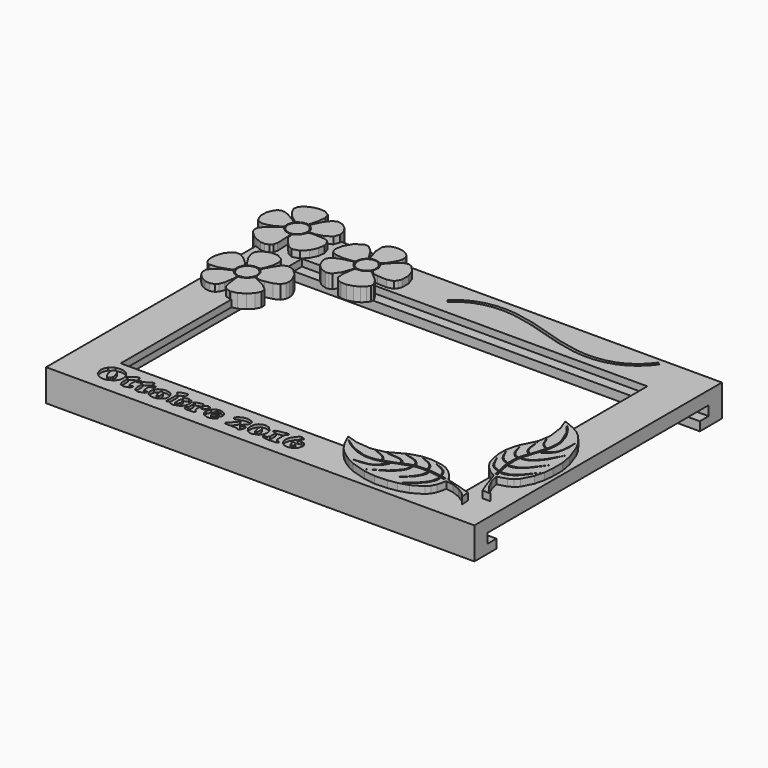
from build123d import *

# Parameters (mm, degrees)
F0_W      = 140.9999974
F0_H      = 92.0000192
F0_W_2    = 7
F1_DEPTH  = 2.5
F2_DEPTH  = 9
F3_DEPTH  = 2.3
F6_DEPTH  = 4
F5_W      = 4
F5_H      = 3.5
F7_DEPTH  = 4
F8_W      = 92.0000192
F8_H      = 3.5
F9_DEPTH  = 4
F11_DEPTH = 1
F12_DEPTH = 2.5
F13_DEPTH = 2.5
F14_DEPTH = 2


# Not quite as in the source:
# - ends of sketch curves that miss each other by under 0.0002 mm in the source are joined


with BuildPart() as f1:
    # F0 (on Top) → F1 (new body)
    with BuildSketch(Plane.XY):
        with Locations((19.9077800781, 3.6383251339)):
            Rectangle(F0_W, F0_H)
        Polygon((-42.5922186219, -37.3616844661), (-42.5922186219, 44.6383347339), (-42.3106248219, 44.6383347339), (82.4077787781, 44.6383347339), (82.4077787781, -37.3616844661), align=None, mode=Mode.SUBTRACT)
        Polygon((90.4077787781, -42.3616844661), (-50.5922186219, -42.3616844661), (-50.5922186219, 49.6383347339), (90.4077787781, 49.6383347339), (97.4077787781, 49.6383347339), (97.4077787781, 59.6383347339), (-57.5922186219, 59.6383347339), (-57.5922186219, -52.2210754661), (-57.5922186219, -52.3616844661), (-57.3105186219, -52.3616844661), (97.4077787781, -52.3616844661), (97.4077787781, -52.2210754661), (97.4077787781, -42.3616844661), align=None)
        with Locations((93.9077787781, 3.6383251339)):
            Rectangle(F0_W_2, F0_H)
    extrude(amount=F1_DEPTH)

    # F0 (on Top) → F2 (join)
    with BuildSketch(Plane.XY):
        Polygon((90.4077787781, -42.3616844661), (-50.5922186219, -42.3616844661), (-50.5922186219, 49.6383347339), (90.4077787781, 49.6383347339), (97.4077787781, 49.6383347339), (97.4077787781, 59.6383347339), (-57.5922186219, 59.6383347339), (-57.5922186219, -52.2210754661), (-57.5922186219, -52.3616844661), (-57.3105186219, -52.3616844661), (97.4077787781, -52.3616844661), (97.4077787781, -52.2210754661), (97.4077787781, -42.3616844661), align=None)
    extrude(amount=-F2_DEPTH)

    # F0 (on Top) → F3 (join)
    with BuildSketch(Plane.XY):
        with Locations((93.9077787781, 3.6383251339)):
            Rectangle(F0_W_2, F0_H)
    extrude(amount=-F3_DEPTH)

    # F4 (on face) → F6 (cut)
    with BuildSketch(Plane(origin=(0, -42.3616844661, 0), x_dir=(-1, 0, 0), z_dir=(0, 1, 0))):
        Polygon((54.5922186219, -2.3), (-97.4077787781, -2.3), (-97.4077787781, -5.8), (54.5728355646, -5.8), (54.5922186219, -5.8), align=None)
    extrude(amount=-F6_DEPTH, mode=Mode.SUBTRACT)

    # F5 (on face) → F7 (cut)
    with BuildSketch(Plane.XZ.offset(-49.6383347339)):
        with Locations((-52.5922186219, -4.05)):
            Rectangle(F5_W, F5_H)
        Polygon((97.4077787781, -5.8), (97.4077787781, -2.3), (90.4077787781, -2.3), (-50.5922186219, -2.3), (-50.5922186219, -5.8), align=None)
    extrude(amount=-F7_DEPTH, mode=Mode.SUBTRACT)

    # F8 (on face) → F9 (cut)
    with BuildSketch(Plane.YZ.offset(-50.5922186219)):
        with Locations((3.6383251339, -4.05)):
            Rectangle(F8_W, F8_H)
    extrude(amount=-F9_DEPTH, mode=Mode.SUBTRACT)

    # F10 (on face) → F11 (cut)
    with BuildSketch(Plane.XY.offset(2.5)):
        Polygon((-39.0562498219, -40.2667686661), (-40.3832982219, -40.0642036661), (-42.0479634219, -40.3508426661), (-43.8284018219, -41.6627272661), (-44.3864906219, -42.7431162661), (-44.5725202219, -43.9778356661), (-43.9937558219, -46.0448876661), (-42.3456260219, -47.4945926661), (-40.5210932219, -47.8914676661), (-39.0714136219, -47.6599466661), (-37.1697156219, -46.4086918661), (-36.5247842219, -45.3145360661), (-36.3098240219, -44.0825598661), (-36.7452816219, -42.3186822661), (-37.9083476219, -40.8744890661), align=None)
        Polygon((-41.6400648219, -42.0596022661), (-40.9069446219, -41.6461918661), (-40.3502274219, -41.8501538661), (-39.8651636219, -42.3793120661), (-39.3084210219, -43.6967084661), (-39.0934608219, -45.1353898661), (-39.3525154219, -45.9622106661), (-40.0250058219, -46.2764086661), (-40.5376286219, -46.1165410661), (-40.9565508219, -45.6865952661), (-41.5959704219, -44.2369156661), (-41.8495386219, -42.7927224661), align=None, mode=Mode.SUBTRACT)
        Polygon((-32.5560342219, -45.5598238661), (-32.5560342219, -43.6967084661), (-32.5009162219, -43.4872600661), (-32.2914678219, -43.4321420661), (-31.2937558219, -43.4321420661), (-31.0126286219, -43.3329042661), (-30.9354634219, -42.9635882661), (-30.9354634219, -42.6383920661), (-30.9960932219, -42.3241940661), (-31.2606850219, -42.2470288661), (-32.2804188219, -42.2470288661), (-32.5064280219, -42.1973972661), (-32.5560342219, -41.9824370661), (-32.5560342219, -41.2382932661), (-32.6056404219, -40.9902368661), (-32.7875552219, -40.9240952661), (-33.2340364219, -40.9240952661), (-33.4655320219, -40.9737014661), (-35.9901142219, -42.5612014661), (-36.1168856219, -42.8037460661), (-36.1168856219, -43.0462906661), (-36.0727912219, -43.2943216661), (-35.8688546219, -43.3439278661), (-35.3010884219, -43.3439278661), (-35.1467580219, -43.3769986661), (-35.1136872219, -43.5313544661), (-35.1136872219, -46.0779584661), (-34.5789918219, -47.3953802661), (-33.1623830219, -47.8914676661), (-31.2661968219, -47.2244890661), (-30.8913690219, -46.5685340661), (-31.0016050219, -46.2212906661), (-31.2441496219, -46.0614230661), (-31.4095036219, -46.1110292661), (-31.9772698219, -46.3094794661), (-32.3961920219, -46.1000056661), align=None)
        Polygon((-27.3305176219, -45.5598238661), (-27.3305176219, -43.6967084661), (-27.2753996219, -43.4872600661), (-27.0659258219, -43.4321420661), (-26.0682392219, -43.4321420661), (-25.7871120219, -43.3329042661), (-25.7099468219, -42.9635882661), (-25.7099468219, -42.6383920661), (-25.7705766219, -42.3241940661), (-26.0351684219, -42.2470288661), (-27.0549022219, -42.2470288661), (-27.2809114219, -42.1973972661), (-27.3305176219, -41.9824370661), (-27.3305176219, -41.2382932661), (-27.3801238219, -40.9902368661), (-27.5620386219, -40.9240952661), (-28.0085198219, -40.9240952661), (-28.2400154219, -40.9737014661), (-30.7645976219, -42.5612014661), (-30.8913690219, -42.8037460661), (-30.8913690219, -43.0462906661), (-30.8472746219, -43.2943216661), (-30.6433126219, -43.3439278661), (-30.0755718219, -43.3439278661), (-29.9212414219, -43.3769986661), (-29.8881452219, -43.5313544661), (-29.8881452219, -46.0779584661), (-29.3534752219, -47.3953802661), (-27.9368664219, -47.8914676661), (-26.0406802219, -47.2244890661), (-25.6658524219, -46.5685340661), (-25.7760884219, -46.2212906661), (-26.0186330219, -46.0614230661), (-26.1839870219, -46.1110292661), (-26.7517532219, -46.3094794661), (-27.1706754219, -46.1000056661), align=None)
        Polygon((-20.2529092219, -42.7706752661), (-22.0223240219, -42.2470288661), (-23.3631392219, -42.4647576661), (-24.4862510219, -43.1179440661), (-25.2138594219, -44.0632812661), (-25.4563786219, -45.2456258661), (-25.2579538219, -46.3039676661), (-24.6626286219, -47.1418120661), (-23.7214316219, -47.7040410661), (-22.5294350219, -47.8914676661), (-21.2547360219, -47.6916458661), (-20.1316496219, -47.0922058661), (-19.3089690219, -46.1647756661), (-19.0347252219, -45.0582246661), (-19.3764822219, -43.7463146661), align=None)
        Polygon((-22.8546566219, -43.7022202661), (-22.4632934219, -43.5203308661), (-21.9561570219, -43.9061822661), (-21.6585198219, -44.8652862661), (-21.5317230219, -45.9181162661), (-21.6543796219, -46.3852730661), (-22.0223240219, -46.5409750661), (-22.5790412219, -46.0889820661), (-22.8767038219, -45.0802718661), (-22.9979634219, -44.1762604661), align=None, mode=Mode.SUBTRACT)
        Polygon((-15.7053948219, -42.6990218661), (-15.6337414219, -40.5492674661), (-15.9203550219, -40.2185340661), (-17.0227912219, -40.3618662661), (-18.0921566219, -40.6870878661), (-18.8803948219, -41.4091590661), (-18.7701334219, -41.7123334661), (-18.3732584219, -41.9493662661), (-18.1252274219, -42.1753500661), (-18.0811330219, -42.8864230661), (-18.0811330219, -44.4077814661), (-18.1197156219, -46.0834702661), (-18.2685342219, -46.9709208661), (-18.2960932219, -47.1363002661), (-17.9543362219, -47.3567722661), (-17.6181164219, -47.3016542661), (-17.2763594219, -47.1969300661), (-17.1440508219, -47.2465362661), (-16.1408524219, -47.7426236661), (-15.1045578219, -47.8914676661), (-13.0871120219, -47.1969300661), (-12.1900094219, -46.0765868661), (-11.8909752219, -44.6337906661), (-12.0756332219, -43.6154030661), (-12.6296072219, -42.8092578661), (-13.9910980219, -42.2525406661), (-15.4132440219, -42.7816988661), (-15.6337414219, -42.9305174661), (-15.7053948219, -42.8202814661), align=None)
        Polygon((-15.5896216219, -44.1156306661), (-15.1596758219, -43.9116940661), (-14.6691002219, -44.1762604661), (-14.3163196219, -45.5763592661), (-14.5257934219, -46.5685340661), (-15.1376286219, -46.9102910661), (-15.6061570219, -46.4913688661), (-15.6943712219, -44.7440266661), align=None, mode=Mode.SUBTRACT)
        Polygon((-8.5616448219, -42.3682884661), (-8.9144254219, -42.2856114661), (-10.3585932219, -42.5446660661), (-11.2626046219, -42.9250056661), (-11.5326828219, -43.3769986661), (-11.1413196219, -43.8235052661), (-10.9208476219, -43.9998828661), (-10.8657296219, -44.3526634661), (-10.9539184219, -46.2102670661), (-11.0365954219, -46.4472744661), (-11.2570928219, -46.6347010661), (-11.5878008219, -47.1473238661), (-11.1358078219, -47.6819938661), (-9.6530320219, -47.8528850661), (-8.0986282219, -47.7426236661), (-7.6741688219, -47.5221516661), (-7.5143266219, -47.1252766661), (-8.0104140219, -46.6071420661), (-8.3080766219, -46.4803452661), (-8.4128008219, -46.2488496661), (-8.4734560219, -45.1133426661), (-8.4293362219, -44.3857342661), (-8.2253996219, -44.2093566661), (-8.0104140219, -44.3251044661), (-7.5143266219, -44.7274912661), (-7.0402864219, -44.8267036661), (-6.1748830219, -44.4904584661), (-5.8606850219, -44.0439772661), (-5.7394254219, -43.5093072661), (-5.8386378219, -43.0297552661), (-6.0922060219, -42.6163194661), (-6.9135150219, -42.2911232661), (-8.0655320219, -42.9801236661), (-8.2750058219, -43.1399912661), (-8.4458716219, -42.8974466661), align=None)
        Polygon((-3.0439774219, -45.2731848661), (-0.4532536219, -45.2731848661), (-0.0674022219, -45.0472010661), (0.0814163781, -44.4573876661), (-0.1776636219, -43.5534016661), (-0.7729634219, -42.8478404661), (-2.5534018219, -42.2525406661), (-3.7715858219, -42.4895480661), (-5.0063052219, -43.4431656661), (-5.5685342219, -45.1078308661), (-5.2433126219, -46.4197154661), (-4.6149420219, -47.2189772661), (-2.6746614219, -47.8914676661), (-0.6517038219, -47.2355126661), (-0.1556164219, -46.4693216661), (-0.2934114219, -46.1055174661), (-0.5745386219, -45.9291398661), (-0.8721758219, -46.0614230661), (-1.4068712219, -46.3149912661), (-1.9911474219, -46.4142036661), (-2.8289918219, -46.1000056661), (-3.2148432219, -45.4220288661), align=None)
        Polygon((-2.3439280219, -44.2424274661), (-2.9006452219, -44.2424274661), (-3.1817724219, -44.1762604661), (-3.2589376219, -43.9447648661), (-3.0935836219, -43.4872600661), (-2.6085198219, -43.2447154661), (-2.1620386219, -43.4321420661), (-1.9911474219, -43.9172058661), align=None, mode=Mode.SUBTRACT)
        Polygon((3.6698267781, -47.7426236661), (7.4236165781, -47.7426236661), (7.7763717781, -47.7867434661), (7.9748219781, -47.9851682661), (8.1622231781, -48.2001538661), (8.3827205781, -48.2607836661), (9.0111165781, -47.9300502661), (9.4355505781, -47.1969300661), (9.5953927781, -46.3590856661), (9.4741331781, -45.7389700661), (9.1103289781, -45.5322648661), (8.9339259781, -45.5708474661), (8.6803831781, -45.7968566661), (7.8149797781, -46.1716590661), (7.4677109781, -46.0669348661), (7.3243787781, -45.8023684661), (7.7984189781, -45.2070432661), (8.7988995781, -44.1183992661), (9.1323761781, -43.1124322661), (8.9339259781, -42.3848238661), (8.4102795781, -41.8446420661), (6.5857467781, -41.4201826661), (5.2008371781, -41.6337966661), (3.9454421781, -42.2745878661), (3.4217703781, -42.7927224661), (3.2233455781, -43.2777862661), (3.4383311781, -43.7187556661), (3.9178831781, -43.9172058661), (4.2375929781, -43.8179934661), (4.8218691781, -43.3714868661), (5.2077205781, -43.2998334661), (5.6376663781, -43.4652128661), (5.7975085781, -43.9006704661), (5.5329421781, -44.6613496661), (3.9564657781, -46.5299514661), (3.2784635781, -47.1969300661), (3.1737393781, -47.4615218661), align=None)
        Polygon((14.5673665781, -41.7509160661), (13.1121497781, -41.3816000661), (11.9807829781, -41.5759100661), (11.0561213781, -42.1588146661), (10.3574435781, -43.2006210661), (10.1245509781, -44.5731354661), (10.3794907781, -45.9911412661), (11.1443101781, -47.0922058661), (12.0951591781, -47.6916458661), (13.2278975781, -47.8914676661), (15.2012489781, -47.1748828661), (16.0487453781, -46.0986340661), (16.3312441781, -44.7550502661), (15.9839753781, -43.2281800661), align=None)
        Polygon((12.6008985781, -43.2419722661), (12.9853783781, -43.0242434661), (13.4869775781, -43.4321420661), (13.7570811781, -44.3526634661), (13.8673171781, -45.4110052661), (13.7419173781, -46.0765868661), (13.3657179781, -46.2984558661), (12.9081877781, -45.9456752661), (12.4727301781, -43.8951586661), align=None, mode=Mode.SUBTRACT)
        Polygon((17.5439163781, -46.7063544661), (17.1801121781, -46.6677718661), (16.8383551781, -46.7945432661), (16.7005601781, -47.0811822661), (17.1249941781, -47.5441988661), (18.3486899781, -47.8143024661), (19.6826217781, -47.8969794661), (21.7772581781, -47.7150646661), (22.5103783781, -47.1638592661), (21.9922183781, -46.7394252661), (21.3528241781, -46.6071420661), (21.1047677781, -46.2047552661), (21.0606733781, -45.9126044661), (21.0110671781, -44.3306162661), (21.0882323781, -42.6549274661), (21.4795955781, -42.2911232661), (21.7662345781, -42.1202320661), (21.8378879781, -41.8942482661), (21.6173905781, -41.5359558661), (20.9228783781, -41.4202080661), (17.6045461781, -42.0816494661), (17.1139705781, -42.3903356661), (16.9375929781, -42.7376044661), (17.0533407781, -43.0077080661), (17.3565151781, -43.1069204661), (17.5494281781, -43.0958714661), (17.7699255781, -43.0793360661), (18.2108949781, -43.1951092661), (18.3321545781, -43.6085196661), (18.2935719781, -45.9897696661), (17.7533901781, -46.7284016661), align=None)
        Polygon((26.1924893781, -40.7422058661), (25.4152747781, -40.5713146661), (24.8364849781, -40.8579536661), (23.9876169781, -41.8336184661), (23.1484009781, -43.2777862661), (22.8686453781, -44.6889086661), (23.0946545781, -45.8740218661), (23.8608455781, -47.0536232661), (24.8943715781, -47.6819938661), (26.2090247781, -47.8914676661), (27.7455469781, -47.5455704661), (28.8493547781, -46.5079042661), (29.3344185781, -44.9314278661), (29.1345967781, -43.9998828661), (28.5351567781, -43.2777862661), (27.2728783781, -42.8368168661), (26.4129613781, -43.0021708661), (26.0160863781, -43.1234558661), (25.8948267781, -43.0683378661), (25.8452205781, -42.9250056661), (26.0160863781, -42.4178946661), (26.4129613781, -41.8446420661), (26.8153481781, -41.3760882661), (26.8815151781, -41.2052224661), (26.6830649781, -40.9681896661), align=None)
        Polygon((25.6302349781, -44.5731354661), (26.0160863781, -44.3967578661), (26.4129613781, -44.5455764661), (26.8153481781, -45.1409016661), (26.9807275781, -45.9070926661), (26.8429071781, -46.2653850661), (26.4791283781, -46.3976682661), (25.8176615781, -45.9511870661), (25.4924399781, -45.0416892661), align=None, mode=Mode.SUBTRACT)
        Polygon((76.7236557781, 57.2223175339), (75.7524359781, 57.8975511339), (73.8715151781, 55.5857955339), (71.6687509781, 53.5751315339), (69.1965689781, 51.9068087339), (66.5074455781, 50.6220513339), (63.2374749781, 49.6519237339), (59.8428157781, 49.1732353339), (56.3862313781, 49.1225369339), (52.9304597781, 49.4364047339), (46.1256219781, 50.8679233339), (39.3970095781, 52.8715769339), (32.6121615781, 54.8672803339), (25.6447383781, 56.2565841339), (22.0671229781, 56.5266877339), (18.4725403781, 56.4069013339), (14.9295197781, 55.8262319339), (11.5066411781, 54.7137373339), (8.1951923781, 52.9586227339), (5.2492241781, 50.6419141339), (6.0611859781, 49.7814637339), (8.8406317781, 51.9669305339), (11.9646793781, 53.6228835339), (15.2065575781, 54.6750785339), (18.5874753781, 55.2281127339), (22.0405037781, 55.3435811339), (25.4986883781, 55.0830533339), (32.3128987781, 53.7218419339), (39.0447877781, 51.7421405339), (45.8184851781, 49.7243137339), (52.7684077781, 48.2645249339), (56.3391651781, 47.9396843339), (59.9332397781, 47.9921353339), (63.4865981781, 48.4944203339), (66.9351815781, 49.5190817339), (69.7845027781, 50.8796073339), (72.4008297781, 52.6446279339), (74.7314575781, 54.7726907339), align=None)
    extrude(amount=-F11_DEPTH, mode=Mode.SUBTRACT)

    # F10 (on face) → F12 (join)
    with BuildSketch(Plane.XY.offset(2.5)):
        Polygon((82.4077787781, -24.8222918728), (82.4077787781, -26.6389711426), (83.5959051781, -27.6658794661), (85.6334931781, -28.8352954661), (87.3536573781, -34.0525824661), (88.8356203781, -37.9930876661), (91.8024165781, -38.0176748661), (90.1737685781, -36.8249162661), (88.5281025781, -34.5089188661), (87.2255143781, -31.6619344661), (86.6260997781, -28.8761386661), (89.8929969781, -27.9246038661), (91.4917237781, -26.9786316661), (92.7525035781, -25.7694392661), (94.7395455781, -21.8603792661), (95.6326857781, -18.3121008661), (95.9526241781, -15.0635424661), (95.9534877781, -10.5948696661), (95.1512541781, -6.4291426661), (93.2918471781, -1.1702758661), (92.0235743781, 1.1986551339), (90.3933007781, 3.4321279339), (88.7402433781, 5.2896553339), (87.1759843781, 6.5801277339), (84.6684455781, 8.0475619339), (82.4077787781, 8.9595404574), (82.4077787781, 8.3104146703), (84.4963351781, 6.1215307339), (86.1499005781, 3.5666209339), (87.1506859781, 1.4285505339), (87.9832979781, -1.5905950661), (88.0010525781, -4.5525652661), (87.3128395781, -8.3344220661), (86.2622701781, -10.8951738661), (84.7916355781, -15.7043590661), (84.5624513781, -18.1463658661), (84.8761921781, -22.3070382661), (86.0933347781, -27.5964866661), (85.3364147781, -27.6957498661), (84.2792921781, -22.8573800661), (83.9435803781, -20.3930720661), (83.9373319781, -17.8612254661), (84.0348171781, -16.1369210661), (84.5069523781, -14.1969706661), (85.9491643781, -10.3173746661), (86.93214141, -6.8113595297), (85.8107597781, -6.3159856661), (84.8599869781, -5.5106532661), (84.1876743781, -4.4411100661), (83.0931883781, -1.6576510661), (83.9026609781, -3.1752502661), (84.6109907781, -4.7800984661), (85.5973489781, -5.8532992661), (86.9969143781, -6.4533996661), (86.9495239967, -6.7493605105), (87.3466469781, -5.3329294661), (87.5562223781, -2.9158908661), (87.3419733781, -0.6577292661), (85.3261531781, 4.3245061339), (82.4077787781, 8.2377713206), (82.4077787781, 4.2659286823), (82.9804377781, 0.0068363339), (82.4077787781, -3.6377173348), (82.4077787781, -14.9819990927), (83.7716985781, -15.8728372661), (83.7145485781, -16.3442358661), (82.4425927781, -15.4811438661), (82.4077787781, -15.4407730706), (82.4077787781, -19.7287612836), (83.6703271781, -20.2725490661), (83.7088589781, -20.6955098661), (82.4077787781, -20.1635944295), (82.4077787781, -24.4548522413), (82.5383761781, -24.5969498661), (84.3776155781, -25.3688558661), (84.3728403781, -25.8263860661), (82.7927063781, -25.1483330661), align=None)
        Polygon((86.3122065781, -26.4910024661), (86.2192425781, -26.0206706661), (88.9610709781, -25.3765266661), (90.9982779781, -23.9398772661), (95.1068295781, -18.9487010661), (91.8285785781, -23.5265430661), (90.3175833781, -25.0708122661), (88.4368403781, -26.0726136661), (87.3511427781, -26.4410660661), align=None, mode=Mode.SUBTRACT)
        Polygon((85.2411647781, -21.7964474661), (85.2425871781, -21.4030268661), (87.9522083781, -20.6377502661), (90.2719395781, -18.7704438661), (94.6556239781, -13.1043134661), (91.1733093781, -18.1236074661), (89.5136225781, -20.0028264661), (87.4600833781, -21.3564686661), (86.3037991781, -21.7672628661), (85.1797729781, -21.8577630661), align=None, mode=Mode.SUBTRACT)
        Polygon((83.7255721781, -10.8170434661), (84.9285669781, -11.8759440661), (84.7747699781, -12.2748256661), (83.7241497781, -11.3737098661), (83.0639783781, -10.0839232661), (82.8124421781, -8.6356406661), (82.4822675781, -5.1122034661), (82.8942555781, -7.2103958661), (83.0841713781, -9.2173514661), align=None, mode=Mode.SUBTRACT)
        Polygon((85.2076367781, -16.1215032661), (85.3454317781, -15.6061880661), (86.4809387781, -15.4454822661), (87.7624449781, -14.9350184661), (89.7831419781, -13.1407624661), (91.1158291781, -11.3798566661), (94.1942329781, -5.9575154661), (91.7894117781, -10.8244348661), (91.2931211781, -11.7546590661), (89.7832181781, -13.7347922661), (88.2971657781, -15.1115484661), (86.8241181781, -15.7740058661), align=None, mode=Mode.SUBTRACT)
        Polygon((87.3097915781, -9.6943888661), (87.4949067781, -9.0630210661), (89.7755473781, -7.2778328661), (90.5238821781, -6.1284828661), (91.0172771781, -4.6301876661), (91.3649269781, 0.9116097339), (91.4948225781, -2.3485564661), (91.1874317781, -4.9346574661), (90.6404935781, -6.5659216661), (89.2364831781, -8.4606346661), align=None, mode=Mode.SUBTRACT)
        Polygon((39.842011439, -37.3616844661), (39.2524704085, -37.3616844661), (40.3360729781, -39.7125152661), (41.9232681781, -42.1460130661), (43.2880101781, -43.6459084661), (45.2234393781, -45.2070432661), (47.5332645781, -46.7271824661), (49.9608695781, -47.8791994661), (55.3036579781, -49.4816346661), (59.5033447781, -50.0810746661), (63.9667597781, -49.8637014661), (67.1959887781, -49.3867402661), (70.6968453781, -48.3227342661), (74.5050165781, -46.1486212661), (75.6517249781, -44.8307422661), (76.5191095781, -43.1880480661), (77.3112593781, -39.8788852661), (80.1228107781, -40.3426130661), (83.0295867781, -41.5057298661), (85.4225969781, -43.0372736661), (86.6928509781, -44.6062062661), (86.5245251781, -41.6441090661), (82.5168623781, -40.3547796661), (77.2223339781, -38.8894282661), (76.2442013792, -37.3616844661), (73.9537955395, -37.3616844661), (74.1559189781, -37.7760446661), (73.6991253781, -37.8029940661), (73.4882151037, -37.3616844661), (64.4903989403, -37.3616844661), (64.6529915781, -37.5779500661), (64.1849203781, -37.6578838661), (63.9702919636, -37.3616844661), (58.6565628279, -37.3616844661), (59.6887647781, -37.8283686661), (60.6397153781, -38.8340816661), (60.2487839781, -39.0070302661), (59.1328095781, -37.8567658661), (57.7008650039, -37.3616844661), (49.6138425534, -37.3616844661), (48.2855363781, -37.6369288661), (45.0622309962, -37.3616844661), (39.8848763277, -37.3616844661), (44.0866115781, -40.1890954661), (49.1606679781, -41.9611518661), (51.4265511781, -42.0657236661), (53.8305849781, -41.7392828661), (55.2260700221, -41.2740153251), (54.9327925781, -41.3356768661), (54.2655853781, -39.9668454661), (53.1458517781, -39.0336494661), (51.5085931781, -38.4038818661), (49.9535289781, -37.6689074661), (52.7867465781, -38.6272494661), (53.8876333781, -39.2469586661), (54.7380761781, -40.1575740661), (55.2872144471, -41.2536292118), (58.7414717781, -40.1019480661), (62.5466457781, -38.4734270661), (64.4614501781, -37.9078960661), (66.1789981781, -37.7269718661), (68.7081523781, -37.6105382661), (71.1858461781, -37.8264382661), (76.0697581781, -38.6478996661), (76.0072741781, -39.4087312661), (70.6650699781, -38.4493224661), (66.4940851781, -38.3375370661), (64.0660483781, -38.6847550661), (59.3337743781, -40.3867074661), (56.8269213781, -41.5601112661), (53.0828597781, -42.4307470661), (50.1235057781, -42.5565024661), (47.0675555781, -41.8711596661), (44.8835365781, -40.9751492661), (42.2514869781, -39.4473138661), align=None)
        Polygon((55.8909059781, -44.0711044661), (57.5634959781, -41.7066438661), (58.1851609781, -41.4911502661), (57.0461741781, -43.4753728661), (55.2217175781, -44.9695278661), (53.6188759781, -45.5948504661), (51.0507073781, -46.0271838661), (47.7880773781, -46.0554032661), (53.3065321781, -45.4396564661), (54.7791733781, -44.8742524661), align=None, mode=Mode.SUBTRACT)
        Polygon((63.8893151781, -40.3846246661), (63.9948267781, -39.2426914661), (64.5028775781, -39.0800806661), (64.2340947781, -40.7114972661), (63.6437987781, -42.2148978661), (62.3406517781, -43.7659234661), (60.4359819781, -45.3699842661), (59.5309037781, -45.9107756661), (54.7862345781, -48.5485656661), (60.0530515781, -45.2110564661), (61.7473077781, -43.7946254661), (63.4415385781, -41.6893464661), align=None, mode=Mode.SUBTRACT)
        Polygon((69.1467595781, -41.6026054661), (69.7798799781, -38.8590752661), (70.1727417781, -38.8386028661), (70.2310347781, -38.7743154661), (70.1950937781, -39.9013896661), (69.8408145781, -41.0762412661), (68.5882389781, -43.1929502661), (66.7916461781, -44.9417148661), (61.9469771781, -48.6631450661), (67.3940579781, -44.0100682661), align=None, mode=Mode.SUBTRACT)
        Polygon((73.9288683781, -42.3806836661), (74.4394337781, -39.6108644661), (74.9137025781, -39.6809176661), (74.9141597781, -40.7210730661), (74.5987425781, -41.8233568661), (73.6892447781, -43.7504040661), (72.2199817781, -45.3344496661), (67.8063761781, -48.8306580661), (72.5925997781, -44.4850990661), align=None, mode=Mode.SUBTRACT)
        Polygon((-12.9422558219, 45.8867801339), (-10.8253944219, 46.4736725339), (-10.0408900219, 47.3849991339), (-9.5741142219, 48.5860889339), (-9.5298166219, 51.4818413339), (-10.5647396219, 54.4096993339), (-12.5510958219, 56.6184071339), (-13.9618880219, 57.1482765339), (-15.4609452219, 56.8088309339), (-17.2068650219, 55.5205175339), (-19.3582704219, 53.2037581339), (-20.0420892219, 52.2600211339), (-19.7511322219, 51.6057171339), (-19.0960408219, 49.9026471339), (-19.2493298219, 48.0996789339), (-19.3409222219, 47.4934571339), (-18.6529124219, 46.8839333339), (-17.7361756219, 46.3085979339), (-16.4363814219, 46.0565791339), align=None)
        Polygon((-45.6112278219, 43.7100763339), (-43.0470470219, 44.4288455339), (-41.2036420219, 46.3593725339), (-40.0380614219, 48.8445593339), (-39.7090298219, 51.3540539339), (-40.3751702219, 53.3576313339), (-41.2208124219, 54.0539469339), (-42.5364562219, 54.4803113339), (-47.0275572219, 54.6075399339), (-48.2771610219, 54.3081247339), (-48.4021544219, 53.6125965339), (-49.2000192219, 52.0704355339), (-50.5825158219, 51.0020607339), (-51.0287430219, 50.6574589339), (-50.9266350219, 49.5753173339), (-50.6253910219, 48.5030055339), (-49.5220658219, 46.9481445339), (-47.4045694219, 44.6375319339), align=None)
        Polygon((-42.5922186219, 32.3775420091), (-42.5922186219, 23.9327596608), (-41.9784944219, 23.6751151339), (-40.8202798219, 23.3489537339), (-39.2281570219, 23.4811861339), (-36.5299150219, 24.0420943339), (-34.6559792219, 24.9394509339), (-33.7853942219, 26.3138957339), (-33.5992884219, 27.7198111339), (-33.8199382219, 29.2090893339), (-35.2165572219, 32.0742855339), (-37.4454072219, 34.1825871339), (-38.7063648219, 34.7257661339), (-39.9766696219, 34.8071731339), (-40.9658472219, 34.3986903339), (-41.9755226219, 33.4303661339), align=None)
        Polygon((-26.7615830219, 49.0437969339), (-26.7513214219, 49.4374715339), (-26.3703722219, 51.0412783339), (-25.4230792219, 52.3593097339), (-25.0174920219, 52.7854455339), (-27.5075302219, 56.7626029339), (-29.5965532219, 58.5955685339), (-30.6243134219, 58.7672725339), (-31.7499398219, 58.4868057339), (-33.9363210219, 56.7792145339), (-35.4245832219, 54.1863063339), (-35.9222200219, 51.4875055339), (-35.7081488219, 50.3419909339), (-35.1366996219, 49.4622873339), (-33.6582926219, 48.8117933339), (-31.0597710219, 48.5155531339), (-28.0792334219, 48.7788749339), align=None)
        Polygon((-16.5280514482, 44.6383347339), (-24.1622243817, 44.6383347339), (-24.2788600219, 44.1817035339), (-24.7316658219, 40.5974079339), (-24.4898578219, 38.2244383339), (-23.5451810219, 37.0614993339), (-21.9679426219, 36.4446857339), (-19.9640350219, 36.4113609339), (-17.7393252219, 36.9989137339), (-16.0075532219, 37.9037125339), (-14.7289680219, 39.0003321339), (-13.9946286219, 40.1855215339), (-13.8956702219, 41.3559789339), (-15.2740774219, 43.5413949339), align=None)
        Polygon((-45.0493544219, 28.8051785339), (-44.3935518219, 29.9630629339), (-43.5239828219, 32.4943761339), (-43.2844100219, 35.0165199339), (-43.5431344219, 36.1768173339), (-44.1697016219, 37.1228911339), (-46.2241806219, 38.2921801339), (-48.8436064219, 38.3639351339), (-51.4237130219, 37.1777551339), (-52.4950088219, 35.8463633339), (-52.6268348219, 34.1469509339), (-51.7846978219, 31.8870367339), (-49.9340284219, 28.8741141339), (-49.3335724219, 28.1330183339), (-48.7411174219, 28.3608817339), (-47.2852148219, 28.9154399339), (-45.7747530219, 28.8153639339), align=None)
        Polygon((-57.5922186219, 59.6383347339), (-50.9054715871, 59.6383347339), (-50.4340782219, 61.3726013339), (-50.0464742219, 64.5712487339), (-50.7474126219, 66.5318239339), (-52.6481708219, 67.6120859339), (-54.3338672219, 67.7605743339), (-56.1619306219, 67.5033231339), (-57.9087648219, 66.8944851339), (-59.3508498219, 65.9881877339), (-60.4002000219, 64.6763285339), (-60.5203166219, 63.2179875339), (-59.6810244219, 61.4789257339), (-57.8520974219, 59.3249041339), (-57.5922186219, 59.1312214795), align=None)
        Polygon((-50.6763180219, 12.9225839339), (-49.1059376219, 13.4136929339), (-48.2846032219, 14.3361701339), (-47.6314676219, 15.8664439339), (-47.0996170219, 19.8809901339), (-47.1866120219, 20.9995299339), (-47.6864586219, 21.2600323339), (-49.1985460219, 22.1203811339), (-50.1070278219, 23.2538053339), (-53.1745350219, 21.8660763339), (-55.4472508219, 20.2756299339), (-56.5987090219, 18.7598341339), (-56.6763060219, 17.2002487339), (-55.7273366219, 15.4783827339), (-54.1916018219, 14.0187209339), (-52.4397384219, 13.1455197339), align=None)
        Polygon((-57.5922186219, 31.4267985945), (-57.5922186219, 21.8893522871), (-55.1119454219, 21.9585069339), (-51.5761892219, 23.1175089339), (-50.3858690219, 23.7181935339), (-50.4540934219, 24.0407481339), (-50.4940222219, 25.6275623339), (-49.9720522219, 27.0809503339), (-49.6713416219, 27.8114035339), (-50.3536872219, 28.6524737339), (-52.9271390219, 30.9995607339), (-54.9885014219, 32.2009807339), (-56.5233726219, 32.1426369339), align=None)
        Polygon((-57.5922186219, 51.3998818667), (-57.5922186219, 42.5509348584), (-55.0931748219, 41.5467583339), (-53.5318876219, 41.4714981339), (-52.1617862219, 41.8799809339), (-51.4085238219, 42.7045157339), (-51.0063148219, 44.1962323339), (-51.2237642219, 49.4341441339), (-51.4301646219, 50.5517187339), (-52.0319668219, 50.6692191339), (-53.7630276219, 51.0756445339), (-55.1487500219, 52.1977403339), (-55.6524320219, 52.6539243339), (-56.5192324219, 52.2027441339), align=None)
        Polygon((-58.3444510219, 51.6291867339), (-57.5922186219, 52.0513407308), (-57.5922186219, 58.3858754724), (-59.6399272219, 59.6188583339), (-61.3068784219, 60.2213971339), (-62.5030406219, 60.3216509339), (-63.4289214219, 59.9007475339), (-64.1911754219, 59.1213993339), (-65.1491618219, 56.8456863339), (-65.2259460219, 54.2112745339), (-64.2704996219, 51.9348757339), (-63.2895262219, 51.1112553339), (-62.0419798219, 50.7892341339), (-60.4271748219, 50.9636051339), align=None)
        Polygon((57.8984965781, -33.8612188661), (57.4105130467, -34.1479347624), (61.1516269781, -34.9136424661), (62.5609713781, -35.4366538661), (63.7292697781, -36.3493012661), (64.4903989403, -37.3616844661), (73.4882151037, -37.3616844661), (72.8390305781, -36.0033278661), (71.5046669781, -34.8912396661), (67.4043703781, -33.0260922661), (71.0767277781, -34.4069632661), (72.3886123781, -35.1454428661), (73.4020723781, -36.2306324661), (73.9537955395, -37.3616844661), (76.2442013792, -37.3616844661), (75.9555851781, -36.9108952661), (74.0932571781, -34.9562128661), (71.9553645781, -33.5183442661), (70.1352259781, -32.8479112661), (65.8778303781, -32.2251540661), (62.6639429781, -32.3724740661), (59.5175941781, -33.2198434661), align=None)
        Polygon((68.9988807781, -37.3614404661), (68.5745483781, -37.3434318661), (67.6951749781, -35.5467882661), (66.3608367781, -34.4347000661), (62.2605147781, -32.5695526661), (65.9328975781, -33.9503982661), (67.2447821781, -34.6889032661), (68.2582421781, -35.7740674661), align=None, mode=Mode.SUBTRACT)
        Polygon((-17.1355418219, 59.4965065339), (-17.1987458467, 59.6383347339), (-26.3000436102, 59.6383347339), (-26.1513480219, 57.3544737339), (-24.7713152219, 53.1033773339), (-23.8809182219, 53.1392675339), (-22.4583404219, 53.2709157339), (-20.6316232219, 52.5433835339), (-19.4514884219, 53.5864091339), (-17.5761048219, 56.7306497339), (-17.1438222219, 58.2442103339), align=None)
        Polygon((-42.5922186219, 23.5646985702), (-42.5922186219, 12.7591575143), (-40.7447402219, 13.1467897339), (-38.4791618219, 14.4738635339), (-36.7853374219, 16.2073373339), (-35.8998934219, 18.0218371339), (-36.0594054219, 19.5918873339), (-38.4518822219, 21.6099427339), align=None)
        Polygon((-24.5177990244, 44.6383347339), (-34.3742825943, 44.6383347339), (-34.3564116219, 43.6538407339), (-33.2915166219, 41.1643359339), (-31.3772456219, 39.3722643339), (-29.1648548219, 38.6178589339), (-28.1191368219, 38.7360959339), (-27.2056766219, 39.2413019339), (-25.6360582219, 41.5119603339), (-24.5358572219, 44.5489875339), align=None)
        Polygon((81.5532879781, -25.9004270661), (82.4077787781, -26.6389711426), (82.4077787781, -24.8222918728), (81.6596885781, -24.1886448661), (80.8585217781, -22.9140728661), (79.3013493781, -19.3129116661), (81.3629657781, -23.3180344661), (82.4077787781, -24.4548522413), (82.4077787781, -20.1635944295), (82.0874753781, -20.0326460661), (80.9544575781, -19.0729578661), (80.1532653781, -17.7983858661), (78.5960929781, -14.1972500661), (80.6577347781, -18.2023728661), (81.8331451781, -19.4812628661), (82.4077787781, -19.7287612836), (82.4077787781, -15.4407730706), (81.4744209781, -14.3584384661), (80.8837185781, -12.9760942661), (79.9376672282, -9.2764421595), (79.6749325781, -9.7777516661), (79.1127543781, -11.4260084661), (78.4188263781, -14.6097460661), (78.4273861781, -17.8269862661), (79.2557055781, -22.0492282661), (80.0135145781, -23.8347212661), align=None)
        Polygon((-22.4276318219, 45.8098181339), (-20.7618744219, 46.5203831339), (-19.8811294219, 47.4809603339), (-19.4427762219, 48.5872065339), (-19.7178074219, 50.8501179339), (-21.2359146219, 52.5361445339), (-22.3514572219, 52.9212593339), (-23.6461206219, 52.8722627339), (-24.9566844219, 52.3235211339), (-25.8678840219, 51.3851943339), (-26.3249570219, 50.1445059339), (-26.2731410219, 48.6887049339), (-25.4701200219, 47.0068439339), (-24.0926780219, 46.0095891339), align=None)
        Polygon((-51.9848244219, 50.9922817339), (-50.8660306219, 51.2243869339), (-49.2983172219, 52.4671581339), (-48.6363932219, 54.2201645339), (-48.9241498219, 56.0613343339), (-50.2055798219, 57.5686211339), (-51.9661808219, 58.1680357339), (-53.6733148219, 57.8231037339), (-55.0039446219, 56.6909241339), (-55.6350838219, 54.9285705339), (-55.4441520219, 53.4076185339), (-54.6840570219, 52.1496327339), (-53.4869296219, 51.2970309339), align=None)
        Polygon((-47.0697720219, 21.4676773339), (-45.1469158219, 21.8082405339), (-43.6980490219, 23.1316059339), (-43.1749614219, 24.9004365339), (-43.5899974219, 26.7058177339), (-44.9555268219, 28.1389365339), (-46.5835144219, 28.6109447339), (-48.1943316219, 28.2676383339), (-49.4921954219, 27.2476251339), (-50.1812720219, 25.6895383339), (-49.9471094219, 23.6860117339), (-48.7898854219, 22.1861671339), align=None)
        Polygon((-40.3657468219, 59.0512953339), (-40.466210318, 59.6383347339), (-50.2205466938, 59.6383347339), (-50.8535592219, 58.3767983339), (-50.2247060219, 57.9356003339), (-49.0452062219, 56.8979849339), (-48.4493730219, 55.5447237339), (-48.1579080219, 54.9530307339), (-47.0107170219, 54.9382987339), (-45.8888498219, 54.9711663339), (-43.2962464219, 55.7267147339), (-41.1317346219, 57.0936665339), align=None)
        Polygon((-50.2205466938, 59.6383347339), (-40.466210318, 59.6383347339), (-40.7251314219, 61.1512911339), (-41.9285834219, 63.0679751339), (-43.6677722219, 64.4552215339), (-45.6344942219, 64.9669045339), (-47.2752834219, 64.3207031339), (-48.9873196219, 62.0960441339), align=None)
        Polygon((-43.0061022219, 12.6723177339), (-42.5922186219, 12.7591575143), (-42.5922186219, 23.5646985702), (-42.6124530219, 23.5742517339), (-42.9796354219, 23.7056205339), (-43.3991926219, 23.0243163339), (-44.4073948219, 21.8642221339), (-45.8610876219, 21.2544443339), (-46.8189216219, 21.0158621339), (-46.7908546219, 20.2254903339), (-46.3150110219, 16.2136111339), (-45.7310904219, 14.1069859339), (-44.8694970219, 13.1921287339), align=None)
        Polygon((-34.3818116219, 45.0531013339), (-34.3742825943, 44.6383347339), (-24.5177990244, 44.6383347339), (-24.3069524219, 45.6815481339), (-24.8960800219, 46.0632339339), (-25.8959256219, 46.9922643339), (-26.5320432219, 48.1481421339), (-26.8018928219, 48.6728299339), (-30.5899980219, 47.7739239339), (-32.6161814219, 46.9845427339), (-33.8409186219, 46.1204601339), align=None)
        Polygon((52.6645217781, -36.7295392661), (49.6138425534, -37.3616844661), (57.7008650039, -37.3616844661), (57.5039329781, -37.2935970661), (55.4901193781, -37.2011664661), (53.3744263781, -36.8913118661), (56.9097507781, -37.0503920661), (58.3684981781, -37.2314432661), (58.6565628279, -37.3616844661), (63.9702919636, -37.3616844661), (63.1382625781, -36.2134366661), (61.6489843781, -35.3247922661), (57.4024240288, -34.1526874842), (56.4019539781, -34.7405160661), align=None)
        Polygon((-26.3000436102, 59.6383347339), (-17.1987458467, 59.6383347339), (-17.7140776219, 60.7947259339), (-18.7420918219, 61.7845385339), (-20.0768110219, 62.4514155339), (-21.5753602219, 62.7808789339), (-23.0949406219, 62.7583491339), (-24.4927534219, 62.3693227339), (-25.6259998219, 61.5992963339), (-26.3518302219, 60.4337411339), align=None)
        Polygon((39.8848763277, -37.3616844661), (39.842011439, -37.3616844661), (42.2514869781, -39.4473138661), (44.8835365781, -40.9751492661), (47.0675555781, -41.8711596661), (50.1235057781, -42.5565024661), (53.0828597781, -42.4307470661), (56.8269213781, -41.5601112661), (59.3337743781, -40.3867074661), (64.0660483781, -38.6847550661), (66.4940851781, -38.3375370661), (70.6650699781, -38.4493224661), (76.0072741781, -39.4087312661), (76.0697581781, -38.6478996661), (71.1858461781, -37.8264382661), (68.7081523781, -37.6105382661), (66.1789981781, -37.7269718661), (64.4614501781, -37.9078960661), (62.5466457781, -38.4734270661), (58.7414717781, -40.1019480661), (55.2872144471, -41.2536292118), (55.2906277781, -41.2604420661), (55.2260700221, -41.2740153251), (53.8305849781, -41.7392828661), (51.4265511781, -42.0657236661), (49.1606679781, -41.9611518661), (44.0866115781, -40.1890954661), align=None)
        Polygon((84.4963351781, 6.1215307339), (82.4077787781, 8.3104146703), (82.4077787781, 8.2377713206), (85.3261531781, 4.3245061339), (87.3419733781, -0.6577292661), (87.5562223781, -2.9158908661), (87.3466469781, -5.3329294661), (86.9495239967, -6.7493605105), (86.9391039781, -6.8144352661), (86.93214141, -6.8113595297), (85.9491643781, -10.3173746661), (84.5069523781, -14.1969706661), (84.0348171781, -16.1369210661), (83.9373319781, -17.8612254661), (83.9435803781, -20.3930720661), (84.2792921781, -22.8573800661), (85.3364147781, -27.6957498661), (86.0933347781, -27.5964866661), (84.8761921781, -22.3070382661), (84.5624513781, -18.1463658661), (84.7916355781, -15.7043590661), (86.2622701781, -10.8951738661), (87.3128395781, -8.3344220661), (88.0010525781, -4.5525652661), (87.9832979781, -1.5905950661), (87.1506859781, 1.4285505339), (86.1499005781, 3.5666209339), align=None)
        Polygon((-58.2787920219, 42.8268167339), (-57.5922186219, 42.5509348584), (-57.5922186219, 51.3998818667), (-59.8762742219, 49.6908365339), (-61.3280112219, 47.6539597339), (-61.3000458219, 46.3648081339), (-60.6974308219, 45.0769773339), align=None)
        Polygon((-58.1418860219, 21.8740265339), (-57.5922186219, 21.8893522871), (-57.5922186219, 31.4267985945), (-57.9660672219, 31.1764209339), (-59.1446272219, 29.4772117339), (-59.8870438219, 27.2198883339), (-60.0405868219, 25.3141771339), (-59.7724898219, 23.7009723339), (-59.1253994219, 22.5107537339), align=None)
        Polygon((82.4077787781, -14.9819990927), (82.4077787781, -3.6377173348), (82.2862811781, -4.4109602661), (80.4806713781, -8.2403658661), (79.9420227603, -9.2681316088), (81.3184903781, -13.4529284661), (82.2782547781, -14.8974010661), align=None)
        Polygon((-23.9569404219, 45.4420261339), (-24.1622243817, 44.6383347339), (-16.5280514482, 44.6383347339), (-18.6118152219, 46.4611503339), (-19.5467384219, 47.0952359339), (-20.0401334219, 46.7408043339), (-21.6145524219, 45.7046875339), (-23.3853388219, 45.5067453339), align=None)
        Polygon((-57.5922186219, 58.3858754724), (-57.5922186219, 52.0513407308), (-55.8576386219, 53.0247897339), (-55.8516950219, 53.5540495339), (-55.9703638219, 54.9021545339), (-55.5557596219, 56.3812473339), (-55.3065602219, 56.9195241339), (-55.8444052219, 57.3334679339), align=None)
        Polygon((-51.1748438219, 58.6473083339), (-50.9054715871, 59.6383347339), (-57.5922186219, 59.6383347339), (-57.5922186219, 59.1312214795), (-55.0601040219, 57.2440853339), (-54.6325966219, 57.5786541339), (-53.3032114219, 58.3267603339), (-51.8725310219, 58.4793635339), (-51.3066698219, 58.4231787339), align=None)
        Polygon((-42.8593156219, 24.0448883339), (-42.5922186219, 23.9327596608), (-42.5922186219, 32.3775420091), (-44.1881420219, 29.6529797339), (-44.6599216219, 28.5487401339), (-44.5085884219, 28.2366757339), (-43.2921824219, 26.7752105339), (-42.8656148219, 24.6392483339), align=None)
        Polygon((64.5028775781, -39.0800806661), (63.9948267781, -39.2426914661), (63.8893151781, -40.3846246661), (63.4415385781, -41.6893464661), (61.7473077781, -43.7946254661), (60.0530515781, -45.2110564661), (54.7862345781, -48.5485656661), (59.5309037781, -45.9107756661), (60.4359819781, -45.3699842661), (62.3406517781, -43.7659234661), (63.6437987781, -42.2148978661), (64.2340947781, -40.7114972661), align=None)
        Polygon((86.4809387781, -15.4454822661), (85.3454317781, -15.6061880661), (85.2076367781, -16.1215032661), (86.8241181781, -15.7740058661), (88.2971657781, -15.1115484661), (89.7832181781, -13.7347922661), (91.2931211781, -11.7546590661), (91.7894117781, -10.8244348661), (94.1942329781, -5.9575154661), (91.1158291781, -11.3798566661), (89.7831419781, -13.1407624661), (87.7624449781, -14.9350184661), align=None)
        Polygon((74.9137025781, -39.6809176661), (74.4394337781, -39.6108644661), (73.9288683781, -42.3806836661), (72.5925997781, -44.4850990661), (67.8063761781, -48.8306580661), (72.2199817781, -45.3344496661), (73.6892447781, -43.7504040661), (74.5987425781, -41.8233568661), (74.9141597781, -40.7210730661), align=None)
        Polygon((88.9610709781, -25.3765266661), (86.2192425781, -26.0206706661), (86.3122065781, -26.4910024661), (87.3511427781, -26.4410660661), (88.4368403781, -26.0726136661), (90.3175833781, -25.0708122661), (91.8285785781, -23.5265430661), (95.1068295781, -18.9487010661), (90.9982779781, -23.9398772661), align=None)
        Polygon((70.1727417781, -38.8386028661), (69.7798799781, -38.8590752661), (69.1467595781, -41.6026054661), (67.3940579781, -44.0100682661), (61.9469771781, -48.6631450661), (66.7916461781, -44.9417148661), (68.5882389781, -43.1929502661), (69.8408145781, -41.0762412661), (70.1950937781, -39.9013896661), (70.2310347781, -38.7743154661), align=None)
        Polygon((87.9522083781, -20.6377502661), (85.2425871781, -21.4030268661), (85.2411647781, -21.7964474661), (85.1797729781, -21.8577630661), (86.3037991781, -21.7672628661), (87.4600833781, -21.3564686661), (89.5136225781, -20.0028264661), (91.1733093781, -18.1236074661), (94.6556239781, -13.1043134661), (90.2719395781, -18.7704438661), align=None)
        Polygon((89.7755473781, -7.2778328661), (87.4949067781, -9.0630210661), (87.3097915781, -9.6943888661), (89.2364831781, -8.4606346661), (90.6404935781, -6.5659216661), (91.1874317781, -4.9346574661), (91.4948225781, -2.3485564661), (91.3649269781, 0.9116097339), (91.0172771781, -4.6301876661), (90.5238821781, -6.1284828661), align=None)
        Polygon((58.1851609781, -41.4911502661), (57.5634959781, -41.7066438661), (55.8909059781, -44.0711044661), (54.7791733781, -44.8742524661), (53.3065321781, -45.4396564661), (47.7880773781, -46.0554032661), (51.0507073781, -46.0271838661), (53.6188759781, -45.5948504661), (55.2217175781, -44.9695278661), (57.0461741781, -43.4753728661), align=None)
        Polygon((82.4077787781, 8.3104146703), (82.4077787781, 8.9595404574), (80.7415039781, 9.6317345339), (81.2410965781, 8.1999619339), (82.2095477781, 5.7402513339), (82.4077787781, 4.2659286823), (82.4077787781, 8.2377713206), (82.1597383781, 8.5703701339), align=None)
        Polygon((38.5634831781, -35.8669552661), (39.2524704085, -37.3616844661), (39.842011439, -37.3616844661), (39.6923099781, -37.2321036661), (39.8848763277, -37.3616844661), (45.0622309962, -37.3616844661), (42.5215143781, -37.1447276661), (40.0177601781, -36.2965962661), align=None)
        Polygon((82.9804377781, 0.0068363339), (82.4077787781, 4.2659286823), (82.4077787781, -3.6377173348), align=None)
        Polygon((67.6951749781, -35.5467882661), (68.5745483781, -37.3434318661), (68.9988807781, -37.3614404661), (68.2582421781, -35.7740674661), (67.2447821781, -34.6889032661), (65.9328975781, -33.9503982661), (62.2605147781, -32.5695526661), (66.3608367781, -34.4347000661), align=None)
        Polygon((72.8390305781, -36.0033278661), (73.4882151037, -37.3616844661), (73.9537955395, -37.3616844661), (73.4020723781, -36.2306324661), (72.3886123781, -35.1454428661), (71.0767277781, -34.4069632661), (67.4043703781, -33.0260922661), (71.5046669781, -34.8912396661), align=None)
        Polygon((84.7747699781, -12.2748256661), (84.9285669781, -11.8759440661), (83.7255721781, -10.8170434661), (83.0841713781, -9.2173514661), (82.8942555781, -7.2103958661), (82.4822675781, -5.1122034661), (82.8124421781, -8.6356406661), (83.0639783781, -10.0839232661), (83.7241497781, -11.3737098661), align=None)
        Polygon((57.4105130467, -34.1479347624), (57.4024240288, -34.1526874842), (61.6489843781, -35.3247922661), (63.1382625781, -36.2134366661), (63.9702919636, -37.3616844661), (64.4903989403, -37.3616844661), (63.7292697781, -36.3493012661), (62.5609713781, -35.4366538661), (61.1516269781, -34.9136424661), align=None)
        Polygon((86.93214141, -6.8113595297), (86.9495239967, -6.7493605105), (86.9969143781, -6.4533996661), (85.5973489781, -5.8532992661), (84.6109907781, -4.7800984661), (83.9026609781, -3.1752502661), (83.0931883781, -1.6576510661), (84.1876743781, -4.4411100661), (84.8599869781, -5.5106532661), (85.8107597781, -6.3159856661), align=None)
        Polygon((54.9327925781, -41.3356768661), (55.2260700221, -41.2740153251), (55.2872144471, -41.2536292118), (54.7380761781, -40.1575740661), (53.8876333781, -39.2469586661), (52.7867465781, -38.6272494661), (49.9535289781, -37.6689074661), (51.5085931781, -38.4038818661), (53.1458517781, -39.0336494661), (54.2655853781, -39.9668454661), align=None)
        Polygon((82.0874753781, -20.0326460661), (82.4077787781, -20.1635944295), (82.4077787781, -19.7287612836), (81.8331451781, -19.4812628661), (80.6577347781, -18.2023728661), (78.5960929781, -14.1972500661), (80.1532653781, -17.7983858661), (80.9544575781, -19.0729578661), align=None)
        Polygon((81.4744209781, -14.3584384661), (82.4077787781, -15.4407730706), (82.4077787781, -14.9819990927), (82.2782547781, -14.8974010661), (81.3184903781, -13.4529284661), (79.9420227603, -9.2681316088), (79.9376672282, -9.2764421595), (80.8837185781, -12.9760942661), align=None)
        Polygon((81.6596885781, -24.1886448661), (82.4077787781, -24.8222918728), (82.4077787781, -24.4548522413), (81.3629657781, -23.3180344661), (79.3013493781, -19.3129116661), (80.8585217781, -22.9140728661), align=None)
        Polygon((58.6565628279, -37.3616844661), (57.7008650039, -37.3616844661), (59.1328095781, -37.8567658661), (60.2487839781, -39.0070302661), (60.6397153781, -38.8340816661), (59.6887647781, -37.8283686661), align=None)
        Polygon((82.4077787781, -24.4548522413), (82.4077787781, -24.8222918728), (82.7927063781, -25.1483330661), (84.3728403781, -25.8263860661), (84.3776409781, -25.3688558661), (82.5383761781, -24.5969498661), align=None)
        Polygon((57.5039329781, -37.2935970661), (57.7008650039, -37.3616844661), (58.6565628279, -37.3616844661), (58.3684981781, -37.2314432661), (56.9097507781, -37.0503920661), (53.3744263781, -36.8913118661), (55.4901193781, -37.2011664661), align=None)
        Polygon((82.4077787781, -14.9819990927), (82.4077787781, -15.4407730706), (82.4425927781, -15.4811438661), (83.7145485781, -16.3442358661), (83.7716985781, -15.8728372661), align=None)
        Polygon((49.6138425534, -37.3616844661), (45.0622309962, -37.3616844661), (48.2855363781, -37.6369288661), align=None)
        Polygon((82.4077787781, -19.7287612836), (82.4077787781, -20.1635944295), (83.7088589781, -20.6955098661), (83.6703271781, -20.2725490661), align=None)
        Polygon((73.9537955395, -37.3616844661), (73.4882151037, -37.3616844661), (73.6991253781, -37.8029940661), (74.1559189781, -37.7760446661), align=None)
        Polygon((64.4903989403, -37.3616844661), (63.9702919636, -37.3616844661), (64.1849203781, -37.6578838661), (64.6529915781, -37.5779500661), align=None)
        Polygon((82.4077787781, 8.2377713206), (82.4077787781, 8.3104146703), (82.1597383781, 8.5703701339), align=None)
        Polygon((39.6923099781, -37.2321036661), (39.842011439, -37.3616844661), (39.8848763277, -37.3616844661), align=None)
        Polygon((57.3125947781, -34.1278934661), (57.4024240288, -34.1526874842), (57.4105130467, -34.1479347624), align=None)
        Polygon((79.9376672282, -9.2764421595), (79.9420227603, -9.2681316088), (79.9129051781, -9.1796070661), align=None)
        Polygon((55.2872144471, -41.2536292118), (55.2260700221, -41.2740153251), (55.2906277781, -41.2604420661), align=None)
        Polygon((86.9391039781, -6.8144352661), (86.9495239967, -6.7493605105), (86.93214141, -6.8113595297), align=None)
    extrude(amount=-F12_DEPTH)

    # F10 (on face) → F13 (join)
    with BuildSketch(Plane.XY.offset(2.5)):
        Polygon((-58.3444510219, 51.6291867339), (-57.5922186219, 52.0513407308), (-57.5922186219, 58.3858754724), (-59.6399272219, 59.6188583339), (-61.3068784219, 60.2213971339), (-62.5030406219, 60.3216509339), (-63.4289214219, 59.9007475339), (-64.1911754219, 59.1213993339), (-65.1491618219, 56.8456863339), (-65.2259460219, 54.2112745339), (-64.2704996219, 51.9348757339), (-63.2895262219, 51.1112553339), (-62.0419798219, 50.7892341339), (-60.4271748219, 50.9636051339), align=None)
        Polygon((-57.5922186219, 58.3858754724), (-57.5922186219, 52.0513407308), (-55.8576386219, 53.0247897339), (-55.8516950219, 53.5540495339), (-55.9703638219, 54.9021545339), (-55.5557596219, 56.3812473339), (-55.3065602219, 56.9195241339), (-55.8444052219, 57.3334679339), align=None)
        Polygon((-57.5922186219, 59.6383347339), (-50.9054715871, 59.6383347339), (-50.4340782219, 61.3726013339), (-50.0464742219, 64.5712487339), (-50.7474126219, 66.5318239339), (-52.6481708219, 67.6120859339), (-54.3338672219, 67.7605743339), (-56.1619306219, 67.5033231339), (-57.9087648219, 66.8944851339), (-59.3508498219, 65.9881877339), (-60.4002000219, 64.6763285339), (-60.5203166219, 63.2179875339), (-59.6810244219, 61.4789257339), (-57.8520974219, 59.3249041339), (-57.5922186219, 59.1312214795), align=None)
        Polygon((-51.1748438219, 58.6473083339), (-50.9054715871, 59.6383347339), (-57.5922186219, 59.6383347339), (-57.5922186219, 59.1312214795), (-55.0601040219, 57.2440853339), (-54.6325966219, 57.5786541339), (-53.3032114219, 58.3267603339), (-51.8725310219, 58.4793635339), (-51.3066698219, 58.4231787339), align=None)
        Polygon((-50.2205466938, 59.6383347339), (-40.466210318, 59.6383347339), (-40.7251314219, 61.1512911339), (-41.9285834219, 63.0679751339), (-43.6677722219, 64.4552215339), (-45.6344942219, 64.9669045339), (-47.2752834219, 64.3207031339), (-48.9873196219, 62.0960441339), align=None)
        Polygon((-40.3657468219, 59.0512953339), (-40.466210318, 59.6383347339), (-50.2205466938, 59.6383347339), (-50.8535592219, 58.3767983339), (-50.2247060219, 57.9356003339), (-49.0452062219, 56.8979849339), (-48.4493730219, 55.5447237339), (-48.1579080219, 54.9530307339), (-47.0107170219, 54.9382987339), (-45.8888498219, 54.9711663339), (-43.2962464219, 55.7267147339), (-41.1317346219, 57.0936665339), align=None)
        Polygon((-51.9848244219, 50.9922817339), (-50.8660306219, 51.2243869339), (-49.2983172219, 52.4671581339), (-48.6363932219, 54.2201645339), (-48.9241498219, 56.0613343339), (-50.2055798219, 57.5686211339), (-51.9661808219, 58.1680357339), (-53.6733148219, 57.8231037339), (-55.0039446219, 56.6909241339), (-55.6350838219, 54.9285705339), (-55.4441520219, 53.4076185339), (-54.6840570219, 52.1496327339), (-53.4869296219, 51.2970309339), align=None)
        Polygon((-57.5922186219, 51.3998818667), (-57.5922186219, 42.5509348584), (-55.0931748219, 41.5467583339), (-53.5318876219, 41.4714981339), (-52.1617862219, 41.8799809339), (-51.4085238219, 42.7045157339), (-51.0063148219, 44.1962323339), (-51.2237642219, 49.4341441339), (-51.4301646219, 50.5517187339), (-52.0319668219, 50.6692191339), (-53.7630276219, 51.0756445339), (-55.1487500219, 52.1977403339), (-55.6524320219, 52.6539243339), (-56.5192324219, 52.2027441339), align=None)
        Polygon((-58.2787920219, 42.8268167339), (-57.5922186219, 42.5509348584), (-57.5922186219, 51.3998818667), (-59.8762742219, 49.6908365339), (-61.3280112219, 47.6539597339), (-61.3000458219, 46.3648081339), (-60.6974308219, 45.0769773339), align=None)
        Polygon((-45.6112278219, 43.7100763339), (-43.0470470219, 44.4288455339), (-41.2036420219, 46.3593725339), (-40.0380614219, 48.8445593339), (-39.7090298219, 51.3540539339), (-40.3751702219, 53.3576313339), (-41.2208124219, 54.0539469339), (-42.5364562219, 54.4803113339), (-47.0275572219, 54.6075399339), (-48.2771610219, 54.3081247339), (-48.4021544219, 53.6125965339), (-49.2000192219, 52.0704355339), (-50.5825158219, 51.0020607339), (-51.0287430219, 50.6574589339), (-50.9266350219, 49.5753173339), (-50.6253910219, 48.5030055339), (-49.5220658219, 46.9481445339), (-47.4045694219, 44.6375319339), align=None)
        Polygon((-26.7615830219, 49.0437969339), (-26.7513214219, 49.4374715339), (-26.3703722219, 51.0412783339), (-25.4230792219, 52.3593097339), (-25.0174920219, 52.7854455339), (-27.5075302219, 56.7626029339), (-29.5965532219, 58.5955685339), (-30.6243134219, 58.7672725339), (-31.7499398219, 58.4868057339), (-33.9363210219, 56.7792145339), (-35.4245832219, 54.1863063339), (-35.9222200219, 51.4875055339), (-35.7081488219, 50.3419909339), (-35.1366996219, 49.4622873339), (-33.6582926219, 48.8117933339), (-31.0597710219, 48.5155531339), (-28.0792334219, 48.7788749339), align=None)
        Polygon((-26.3000436102, 59.6383347339), (-17.1987458467, 59.6383347339), (-17.7140776219, 60.7947259339), (-18.7420918219, 61.7845385339), (-20.0768110219, 62.4514155339), (-21.5753602219, 62.7808789339), (-23.0949406219, 62.7583491339), (-24.4927534219, 62.3693227339), (-25.6259998219, 61.5992963339), (-26.3518302219, 60.4337411339), align=None)
        Polygon((-17.1355418219, 59.4965065339), (-17.1987458467, 59.6383347339), (-26.3000436102, 59.6383347339), (-26.1513480219, 57.3544737339), (-24.7713152219, 53.1033773339), (-23.8809182219, 53.1392675339), (-22.4583404219, 53.2709157339), (-20.6316232219, 52.5433835339), (-19.4514884219, 53.5864091339), (-17.5761048219, 56.7306497339), (-17.1438222219, 58.2442103339), align=None)
        Polygon((-12.9422558219, 45.8867801339), (-10.8253944219, 46.4736725339), (-10.0408900219, 47.3849991339), (-9.5741142219, 48.5860889339), (-9.5298166219, 51.4818413339), (-10.5647396219, 54.4096993339), (-12.5510958219, 56.6184071339), (-13.9618880219, 57.1482765339), (-15.4609452219, 56.8088309339), (-17.2068650219, 55.5205175339), (-19.3582704219, 53.2037581339), (-20.0420892219, 52.2600211339), (-19.7511322219, 51.6057171339), (-19.0960408219, 49.9026471339), (-19.2493298219, 48.0996789339), (-19.3409222219, 47.4934571339), (-18.6529124219, 46.8839333339), (-17.7361756219, 46.3085979339), (-16.4363814219, 46.0565791339), align=None)
        Polygon((-22.4276318219, 45.8098181339), (-20.7618744219, 46.5203831339), (-19.8811294219, 47.4809603339), (-19.4427762219, 48.5872065339), (-19.7178074219, 50.8501179339), (-21.2359146219, 52.5361445339), (-22.3514572219, 52.9212593339), (-23.6461206219, 52.8722627339), (-24.9566844219, 52.3235211339), (-25.8678840219, 51.3851943339), (-26.3249570219, 50.1445059339), (-26.2731410219, 48.6887049339), (-25.4701200219, 47.0068439339), (-24.0926780219, 46.0095891339), align=None)
        Polygon((-16.5280514482, 44.6383347339), (-24.1622243817, 44.6383347339), (-24.2788600219, 44.1817035339), (-24.7316658219, 40.5974079339), (-24.4898578219, 38.2244383339), (-23.5451810219, 37.0614993339), (-21.9679426219, 36.4446857339), (-19.9640350219, 36.4113609339), (-17.7393252219, 36.9989137339), (-16.0075532219, 37.9037125339), (-14.7289680219, 39.0003321339), (-13.9946286219, 40.1855215339), (-13.8956702219, 41.3559789339), (-15.2740774219, 43.5413949339), align=None)
        Polygon((-23.9569404219, 45.4420261339), (-24.1622243817, 44.6383347339), (-16.5280514482, 44.6383347339), (-18.6118152219, 46.4611503339), (-19.5467384219, 47.0952359339), (-20.0401334219, 46.7408043339), (-21.6145524219, 45.7046875339), (-23.3853388219, 45.5067453339), align=None)
        Polygon((-24.5177990244, 44.6383347339), (-34.3742825943, 44.6383347339), (-34.3564116219, 43.6538407339), (-33.2915166219, 41.1643359339), (-31.3772456219, 39.3722643339), (-29.1648548219, 38.6178589339), (-28.1191368219, 38.7360959339), (-27.2056766219, 39.2413019339), (-25.6360582219, 41.5119603339), (-24.5358572219, 44.5489875339), align=None)
        Polygon((-34.3818116219, 45.0531013339), (-34.3742825943, 44.6383347339), (-24.5177990244, 44.6383347339), (-24.3069524219, 45.6815481339), (-24.8960800219, 46.0632339339), (-25.8959256219, 46.9922643339), (-26.5320432219, 48.1481421339), (-26.8018928219, 48.6728299339), (-30.5899980219, 47.7739239339), (-32.6161814219, 46.9845427339), (-33.8409186219, 46.1204601339), align=None)
        Polygon((-45.0493544219, 28.8051785339), (-44.3935518219, 29.9630629339), (-43.5239828219, 32.4943761339), (-43.2844100219, 35.0165199339), (-43.5431344219, 36.1768173339), (-44.1697016219, 37.1228911339), (-46.2241806219, 38.2921801339), (-48.8436064219, 38.3639351339), (-51.4237130219, 37.1777551339), (-52.4950088219, 35.8463633339), (-52.6268348219, 34.1469509339), (-51.7846978219, 31.8870367339), (-49.9340284219, 28.8741141339), (-49.3335724219, 28.1330183339), (-48.7411174219, 28.3608817339), (-47.2852148219, 28.9154399339), (-45.7747530219, 28.8153639339), align=None)
        Polygon((-57.5922186219, 31.4267985945), (-57.5922186219, 21.8893522871), (-55.1119454219, 21.9585069339), (-51.5761892219, 23.1175089339), (-50.3858690219, 23.7181935339), (-50.4540934219, 24.0407481339), (-50.4940222219, 25.6275623339), (-49.9720522219, 27.0809503339), (-49.6713416219, 27.8114035339), (-50.3536872219, 28.6524737339), (-52.9271390219, 30.9995607339), (-54.9885014219, 32.2009807339), (-56.5233726219, 32.1426369339), align=None)
        Polygon((-58.1418860219, 21.8740265339), (-57.5922186219, 21.8893522871), (-57.5922186219, 31.4267985945), (-57.9660672219, 31.1764209339), (-59.1446272219, 29.4772117339), (-59.8870438219, 27.2198883339), (-60.0405868219, 25.3141771339), (-59.7724898219, 23.7009723339), (-59.1253994219, 22.5107537339), align=None)
        Polygon((-47.0697720219, 21.4676773339), (-45.1469158219, 21.8082405339), (-43.6980490219, 23.1316059339), (-43.1749614219, 24.9004365339), (-43.5899974219, 26.7058177339), (-44.9555268219, 28.1389365339), (-46.5835144219, 28.6109447339), (-48.1943316219, 28.2676383339), (-49.4921954219, 27.2476251339), (-50.1812720219, 25.6895383339), (-49.9471094219, 23.6860117339), (-48.7898854219, 22.1861671339), align=None)
        Polygon((-42.5922186219, 32.3775420091), (-42.5922186219, 23.9327596608), (-41.9784944219, 23.6751151339), (-40.8202798219, 23.3489537339), (-39.2281570219, 23.4811861339), (-36.5299150219, 24.0420943339), (-34.6559792219, 24.9394509339), (-33.7853942219, 26.3138957339), (-33.5992884219, 27.7198111339), (-33.8199382219, 29.2090893339), (-35.2165572219, 32.0742855339), (-37.4454072219, 34.1825871339), (-38.7063648219, 34.7257661339), (-39.9766696219, 34.8071731339), (-40.9658472219, 34.3986903339), (-41.9755226219, 33.4303661339), align=None)
        Polygon((-42.8593156219, 24.0448883339), (-42.5922186219, 23.9327596608), (-42.5922186219, 32.3775420091), (-44.1881420219, 29.6529797339), (-44.6599216219, 28.5487401339), (-44.5085884219, 28.2366757339), (-43.2921824219, 26.7752105339), (-42.8656148219, 24.6392483339), align=None)
        Polygon((-42.5922186219, 23.5646985702), (-42.5922186219, 12.7591575143), (-40.7447402219, 13.1467897339), (-38.4791618219, 14.4738635339), (-36.7853374219, 16.2073373339), (-35.8998934219, 18.0218371339), (-36.0594054219, 19.5918873339), (-38.4518822219, 21.6099427339), align=None)
        Polygon((-43.0061022219, 12.6723177339), (-42.5922186219, 12.7591575143), (-42.5922186219, 23.5646985702), (-42.6124530219, 23.5742517339), (-42.9796354219, 23.7056205339), (-43.3991926219, 23.0243163339), (-44.4073948219, 21.8642221339), (-45.8610876219, 21.2544443339), (-46.8189216219, 21.0158621339), (-46.7908546219, 20.2254903339), (-46.3150110219, 16.2136111339), (-45.7310904219, 14.1069859339), (-44.8694970219, 13.1921287339), align=None)
        Polygon((-50.6763180219, 12.9225839339), (-49.1059376219, 13.4136929339), (-48.2846032219, 14.3361701339), (-47.6314676219, 15.8664439339), (-47.0996170219, 19.8809901339), (-47.1866120219, 20.9995299339), (-47.6864586219, 21.2600323339), (-49.1985460219, 22.1203811339), (-50.1070278219, 23.2538053339), (-53.1745350219, 21.8660763339), (-55.4472508219, 20.2756299339), (-56.5987090219, 18.7598341339), (-56.6763060219, 17.2002487339), (-55.7273366219, 15.4783827339), (-54.1916018219, 14.0187209339), (-52.4397384219, 13.1455197339), align=None)
        Polygon((82.4077787781, -24.8222918728), (82.4077787781, -26.6389711426), (83.5959051781, -27.6658794661), (85.6334931781, -28.8352954661), (87.3536573781, -34.0525824661), (88.8356203781, -37.9930876661), (91.8024165781, -38.0176748661), (90.1737685781, -36.8249162661), (88.5281025781, -34.5089188661), (87.2255143781, -31.6619344661), (86.6260997781, -28.8761386661), (89.8929969781, -27.9246038661), (91.4917237781, -26.9786316661), (92.7525035781, -25.7694392661), (94.7395455781, -21.8603792661), (95.6326857781, -18.3121008661), (95.9526241781, -15.0635424661), (95.9534877781, -10.5948696661), (95.1512541781, -6.4291426661), (93.2918471781, -1.1702758661), (92.0235743781, 1.1986551339), (90.3933007781, 3.4321279339), (88.7402433781, 5.2896553339), (87.1759843781, 6.5801277339), (84.6684455781, 8.0475619339), (82.4077787781, 8.9595404574), (82.4077787781, 8.3104146703), (84.4963351781, 6.1215307339), (86.1499005781, 3.5666209339), (87.1506859781, 1.4285505339), (87.9832979781, -1.5905950661), (88.0010525781, -4.5525652661), (87.3128395781, -8.3344220661), (86.2622701781, -10.8951738661), (84.7916355781, -15.7043590661), (84.5624513781, -18.1463658661), (84.8761921781, -22.3070382661), (86.0933347781, -27.5964866661), (85.3364147781, -27.6957498661), (84.2792921781, -22.8573800661), (83.9435803781, -20.3930720661), (83.9373319781, -17.8612254661), (84.0348171781, -16.1369210661), (84.5069523781, -14.1969706661), (85.9491643781, -10.3173746661), (86.93214141, -6.8113595297), (85.8107597781, -6.3159856661), (84.8599869781, -5.5106532661), (84.1876743781, -4.4411100661), (83.0931883781, -1.6576510661), (83.9026609781, -3.1752502661), (84.6109907781, -4.7800984661), (85.5973489781, -5.8532992661), (86.9969143781, -6.4533996661), (86.9495239967, -6.7493605105), (87.3466469781, -5.3329294661), (87.5562223781, -2.9158908661), (87.3419733781, -0.6577292661), (85.3261531781, 4.3245061339), (82.4077787781, 8.2377713206), (82.4077787781, 4.2659286823), (82.9804377781, 0.0068363339), (82.4077787781, -3.6377173348), (82.4077787781, -14.9819990927), (83.7716985781, -15.8728372661), (83.7145485781, -16.3442358661), (82.4425927781, -15.4811438661), (82.4077787781, -15.4407730706), (82.4077787781, -19.7287612836), (83.6703271781, -20.2725490661), (83.7088589781, -20.6955098661), (82.4077787781, -20.1635944295), (82.4077787781, -24.4548522413), (82.5383761781, -24.5969498661), (84.3776155781, -25.3688558661), (84.3728403781, -25.8263860661), (82.7927063781, -25.1483330661), align=None)
        Polygon((86.3122065781, -26.4910024661), (86.2192425781, -26.0206706661), (88.9610709781, -25.3765266661), (90.9982779781, -23.9398772661), (95.1068295781, -18.9487010661), (91.8285785781, -23.5265430661), (90.3175833781, -25.0708122661), (88.4368403781, -26.0726136661), (87.3511427781, -26.4410660661), align=None, mode=Mode.SUBTRACT)
        Polygon((85.2411647781, -21.7964474661), (85.2425871781, -21.4030268661), (87.9522083781, -20.6377502661), (90.2719395781, -18.7704438661), (94.6556239781, -13.1043134661), (91.1733093781, -18.1236074661), (89.5136225781, -20.0028264661), (87.4600833781, -21.3564686661), (86.3037991781, -21.7672628661), (85.1797729781, -21.8577630661), align=None, mode=Mode.SUBTRACT)
        Polygon((83.7255721781, -10.8170434661), (84.9285669781, -11.8759440661), (84.7747699781, -12.2748256661), (83.7241497781, -11.3737098661), (83.0639783781, -10.0839232661), (82.8124421781, -8.6356406661), (82.4822675781, -5.1122034661), (82.8942555781, -7.2103958661), (83.0841713781, -9.2173514661), align=None, mode=Mode.SUBTRACT)
        Polygon((85.2076367781, -16.1215032661), (85.3454317781, -15.6061880661), (86.4809387781, -15.4454822661), (87.7624449781, -14.9350184661), (89.7831419781, -13.1407624661), (91.1158291781, -11.3798566661), (94.1942329781, -5.9575154661), (91.7894117781, -10.8244348661), (91.2931211781, -11.7546590661), (89.7832181781, -13.7347922661), (88.2971657781, -15.1115484661), (86.8241181781, -15.7740058661), align=None, mode=Mode.SUBTRACT)
        Polygon((87.3097915781, -9.6943888661), (87.4949067781, -9.0630210661), (89.7755473781, -7.2778328661), (90.5238821781, -6.1284828661), (91.0172771781, -4.6301876661), (91.3649269781, 0.9116097339), (91.4948225781, -2.3485564661), (91.1874317781, -4.9346574661), (90.6404935781, -6.5659216661), (89.2364831781, -8.4606346661), align=None, mode=Mode.SUBTRACT)
        Polygon((81.5532879781, -25.9004270661), (82.4077787781, -26.6389711426), (82.4077787781, -24.8222918728), (81.6596885781, -24.1886448661), (80.8585217781, -22.9140728661), (79.3013493781, -19.3129116661), (81.3629657781, -23.3180344661), (82.4077787781, -24.4548522413), (82.4077787781, -20.1635944295), (82.0874753781, -20.0326460661), (80.9544575781, -19.0729578661), (80.1532653781, -17.7983858661), (78.5960929781, -14.1972500661), (80.6577347781, -18.2023728661), (81.8331451781, -19.4812628661), (82.4077787781, -19.7287612836), (82.4077787781, -15.4407730706), (81.4744209781, -14.3584384661), (80.8837185781, -12.9760942661), (79.9376672282, -9.2764421595), (79.6749325781, -9.7777516661), (79.1127543781, -11.4260084661), (78.4188263781, -14.6097460661), (78.4273861781, -17.8269862661), (79.2557055781, -22.0492282661), (80.0135145781, -23.8347212661), align=None)
        Polygon((82.4077787781, -14.9819990927), (82.4077787781, -3.6377173348), (82.2862811781, -4.4109602661), (80.4806713781, -8.2403658661), (79.9420227603, -9.2681316088), (81.3184903781, -13.4529284661), (82.2782547781, -14.8974010661), align=None)
        Polygon((82.4077787781, 8.3104146703), (82.4077787781, 8.9595404574), (80.7415039781, 9.6317345339), (81.2410965781, 8.1999619339), (82.2095477781, 5.7402513339), (82.4077787781, 4.2659286823), (82.4077787781, 8.2377713206), (82.1597383781, 8.5703701339), align=None)
        Polygon((39.842011439, -37.3616844661), (39.2524704085, -37.3616844661), (40.3360729781, -39.7125152661), (41.9232681781, -42.1460130661), (43.2880101781, -43.6459084661), (45.2234393781, -45.2070432661), (47.5332645781, -46.7271824661), (49.9608695781, -47.8791994661), (55.3036579781, -49.4816346661), (59.5033447781, -50.0810746661), (63.9667597781, -49.8637014661), (67.1959887781, -49.3867402661), (70.6968453781, -48.3227342661), (74.5050165781, -46.1486212661), (75.6517249781, -44.8307422661), (76.5191095781, -43.1880480661), (77.3112593781, -39.8788852661), (80.1228107781, -40.3426130661), (83.0295867781, -41.5057298661), (85.4225969781, -43.0372736661), (86.6928509781, -44.6062062661), (86.5245251781, -41.6441090661), (82.5168623781, -40.3547796661), (77.2223339781, -38.8894282661), (76.2442013792, -37.3616844661), (73.9537955395, -37.3616844661), (74.1559189781, -37.7760446661), (73.6991253781, -37.8029940661), (73.4882151037, -37.3616844661), (64.4903989403, -37.3616844661), (64.6529915781, -37.5779500661), (64.1849203781, -37.6578838661), (63.9702919636, -37.3616844661), (58.6565628279, -37.3616844661), (59.6887647781, -37.8283686661), (60.6397153781, -38.8340816661), (60.2487839781, -39.0070302661), (59.1328095781, -37.8567658661), (57.7008650039, -37.3616844661), (49.6138425534, -37.3616844661), (48.2855363781, -37.6369288661), (45.0622309962, -37.3616844661), (39.8848763277, -37.3616844661), (44.0866115781, -40.1890954661), (49.1606679781, -41.9611518661), (51.4265511781, -42.0657236661), (53.8305849781, -41.7392828661), (55.2260700221, -41.2740153251), (54.9327925781, -41.3356768661), (54.2655853781, -39.9668454661), (53.1458517781, -39.0336494661), (51.5085931781, -38.4038818661), (49.9535289781, -37.6689074661), (52.7867465781, -38.6272494661), (53.8876333781, -39.2469586661), (54.7380761781, -40.1575740661), (55.2872144471, -41.2536292118), (58.7414717781, -40.1019480661), (62.5466457781, -38.4734270661), (64.4614501781, -37.9078960661), (66.1789981781, -37.7269718661), (68.7081523781, -37.6105382661), (71.1858461781, -37.8264382661), (76.0697581781, -38.6478996661), (76.0072741781, -39.4087312661), (70.6650699781, -38.4493224661), (66.4940851781, -38.3375370661), (64.0660483781, -38.6847550661), (59.3337743781, -40.3867074661), (56.8269213781, -41.5601112661), (53.0828597781, -42.4307470661), (50.1235057781, -42.5565024661), (47.0675555781, -41.8711596661), (44.8835365781, -40.9751492661), (42.2514869781, -39.4473138661), align=None)
        Polygon((55.8909059781, -44.0711044661), (57.5634959781, -41.7066438661), (58.1851609781, -41.4911502661), (57.0461741781, -43.4753728661), (55.2217175781, -44.9695278661), (53.6188759781, -45.5948504661), (51.0507073781, -46.0271838661), (47.7880773781, -46.0554032661), (53.3065321781, -45.4396564661), (54.7791733781, -44.8742524661), align=None, mode=Mode.SUBTRACT)
        Polygon((63.8893151781, -40.3846246661), (63.9948267781, -39.2426914661), (64.5028775781, -39.0800806661), (64.2340947781, -40.7114972661), (63.6437987781, -42.2148978661), (62.3406517781, -43.7659234661), (60.4359819781, -45.3699842661), (59.5309037781, -45.9107756661), (54.7862345781, -48.5485656661), (60.0530515781, -45.2110564661), (61.7473077781, -43.7946254661), (63.4415385781, -41.6893464661), align=None, mode=Mode.SUBTRACT)
        Polygon((69.1467595781, -41.6026054661), (69.7798799781, -38.8590752661), (70.1727417781, -38.8386028661), (70.2310347781, -38.7743154661), (70.1950937781, -39.9013896661), (69.8408145781, -41.0762412661), (68.5882389781, -43.1929502661), (66.7916461781, -44.9417148661), (61.9469771781, -48.6631450661), (67.3940579781, -44.0100682661), align=None, mode=Mode.SUBTRACT)
        Polygon((73.9288683781, -42.3806836661), (74.4394337781, -39.6108644661), (74.9137025781, -39.6809176661), (74.9141597781, -40.7210730661), (74.5987425781, -41.8233568661), (73.6892447781, -43.7504040661), (72.2199817781, -45.3344496661), (67.8063761781, -48.8306580661), (72.5925997781, -44.4850990661), align=None, mode=Mode.SUBTRACT)
        Polygon((57.8984965781, -33.8612188661), (57.4105130467, -34.1479347624), (61.1516269781, -34.9136424661), (62.5609713781, -35.4366538661), (63.7292697781, -36.3493012661), (64.4903989403, -37.3616844661), (73.4882151037, -37.3616844661), (72.8390305781, -36.0033278661), (71.5046669781, -34.8912396661), (67.4043703781, -33.0260922661), (71.0767277781, -34.4069632661), (72.3886123781, -35.1454428661), (73.4020723781, -36.2306324661), (73.9537955395, -37.3616844661), (76.2442013792, -37.3616844661), (75.9555851781, -36.9108952661), (74.0932571781, -34.9562128661), (71.9553645781, -33.5183442661), (70.1352259781, -32.8479112661), (65.8778303781, -32.2251540661), (62.6639429781, -32.3724740661), (59.5175941781, -33.2198434661), align=None)
        Polygon((68.9988807781, -37.3614404661), (68.5745483781, -37.3434318661), (67.6951749781, -35.5467882661), (66.3608367781, -34.4347000661), (62.2605147781, -32.5695526661), (65.9328975781, -33.9503982661), (67.2447821781, -34.6889032661), (68.2582421781, -35.7740674661), align=None, mode=Mode.SUBTRACT)
        Polygon((52.6645217781, -36.7295392661), (49.6138425534, -37.3616844661), (57.7008650039, -37.3616844661), (57.5039329781, -37.2935970661), (55.4901193781, -37.2011664661), (53.3744263781, -36.8913118661), (56.9097507781, -37.0503920661), (58.3684981781, -37.2314432661), (58.6565628279, -37.3616844661), (63.9702919636, -37.3616844661), (63.1382625781, -36.2134366661), (61.6489843781, -35.3247922661), (57.4024240288, -34.1526874842), (56.4019539781, -34.7405160661), align=None)
        Polygon((38.5634831781, -35.8669552661), (39.2524704085, -37.3616844661), (39.842011439, -37.3616844661), (39.6923099781, -37.2321036661), (39.8848763277, -37.3616844661), (45.0622309962, -37.3616844661), (42.5215143781, -37.1447276661), (40.0177601781, -36.2965962661), align=None)
    extrude(amount=F13_DEPTH)

    # F10 (on face) → F14 (join)
    with BuildSketch(Plane.XY.offset(2.5)):
        Polygon((39.8848763277, -37.3616844661), (39.842011439, -37.3616844661), (42.2514869781, -39.4473138661), (44.8835365781, -40.9751492661), (47.0675555781, -41.8711596661), (50.1235057781, -42.5565024661), (53.0828597781, -42.4307470661), (56.8269213781, -41.5601112661), (59.3337743781, -40.3867074661), (64.0660483781, -38.6847550661), (66.4940851781, -38.3375370661), (70.6650699781, -38.4493224661), (76.0072741781, -39.4087312661), (76.0697581781, -38.6478996661), (71.1858461781, -37.8264382661), (68.7081523781, -37.6105382661), (66.1789981781, -37.7269718661), (64.4614501781, -37.9078960661), (62.5466457781, -38.4734270661), (58.7414717781, -40.1019480661), (55.2872144471, -41.2536292118), (55.2906277781, -41.2604420661), (55.2260700221, -41.2740153251), (53.8305849781, -41.7392828661), (51.4265511781, -42.0657236661), (49.1606679781, -41.9611518661), (44.0866115781, -40.1890954661), align=None)
        Polygon((54.9327925781, -41.3356768661), (55.2260700221, -41.2740153251), (55.2872144471, -41.2536292118), (54.7380761781, -40.1575740661), (53.8876333781, -39.2469586661), (52.7867465781, -38.6272494661), (49.9535289781, -37.6689074661), (51.5085931781, -38.4038818661), (53.1458517781, -39.0336494661), (54.2655853781, -39.9668454661), align=None)
        Polygon((58.1851609781, -41.4911502661), (57.5634959781, -41.7066438661), (55.8909059781, -44.0711044661), (54.7791733781, -44.8742524661), (53.3065321781, -45.4396564661), (47.7880773781, -46.0554032661), (51.0507073781, -46.0271838661), (53.6188759781, -45.5948504661), (55.2217175781, -44.9695278661), (57.0461741781, -43.4753728661), align=None)
        Polygon((58.6565628279, -37.3616844661), (57.7008650039, -37.3616844661), (59.1328095781, -37.8567658661), (60.2487839781, -39.0070302661), (60.6397153781, -38.8340816661), (59.6887647781, -37.8283686661), align=None)
        Polygon((57.5039329781, -37.2935970661), (57.7008650039, -37.3616844661), (58.6565628279, -37.3616844661), (58.3684981781, -37.2314432661), (56.9097507781, -37.0503920661), (53.3744263781, -36.8913118661), (55.4901193781, -37.2011664661), align=None)
        Polygon((57.4105130467, -34.1479347624), (57.4024240288, -34.1526874842), (61.6489843781, -35.3247922661), (63.1382625781, -36.2134366661), (63.9702919636, -37.3616844661), (64.4903989403, -37.3616844661), (63.7292697781, -36.3493012661), (62.5609713781, -35.4366538661), (61.1516269781, -34.9136424661), align=None)
        Polygon((64.4903989403, -37.3616844661), (63.9702919636, -37.3616844661), (64.1849203781, -37.6578838661), (64.6529915781, -37.5779500661), align=None)
        Polygon((64.5028775781, -39.0800806661), (63.9948267781, -39.2426914661), (63.8893151781, -40.3846246661), (63.4415385781, -41.6893464661), (61.7473077781, -43.7946254661), (60.0530515781, -45.2110564661), (54.7862345781, -48.5485656661), (59.5309037781, -45.9107756661), (60.4359819781, -45.3699842661), (62.3406517781, -43.7659234661), (63.6437987781, -42.2148978661), (64.2340947781, -40.7114972661), align=None)
        Polygon((70.1727417781, -38.8386028661), (69.7798799781, -38.8590752661), (69.1467595781, -41.6026054661), (67.3940579781, -44.0100682661), (61.9469771781, -48.6631450661), (66.7916461781, -44.9417148661), (68.5882389781, -43.1929502661), (69.8408145781, -41.0762412661), (70.1950937781, -39.9013896661), (70.2310347781, -38.7743154661), align=None)
        Polygon((67.6951749781, -35.5467882661), (68.5745483781, -37.3434318661), (68.9988807781, -37.3614404661), (68.2582421781, -35.7740674661), (67.2447821781, -34.6889032661), (65.9328975781, -33.9503982661), (62.2605147781, -32.5695526661), (66.3608367781, -34.4347000661), align=None)
        Polygon((73.9537955395, -37.3616844661), (73.4882151037, -37.3616844661), (73.6991253781, -37.8029940661), (74.1559189781, -37.7760446661), align=None)
        Polygon((72.8390305781, -36.0033278661), (73.4882151037, -37.3616844661), (73.9537955395, -37.3616844661), (73.4020723781, -36.2306324661), (72.3886123781, -35.1454428661), (71.0767277781, -34.4069632661), (67.4043703781, -33.0260922661), (71.5046669781, -34.8912396661), align=None)
        Polygon((74.9137025781, -39.6809176661), (74.4394337781, -39.6108644661), (73.9288683781, -42.3806836661), (72.5925997781, -44.4850990661), (67.8063761781, -48.8306580661), (72.2199817781, -45.3344496661), (73.6892447781, -43.7504040661), (74.5987425781, -41.8233568661), (74.9141597781, -40.7210730661), align=None)
        Polygon((84.4963351781, 6.1215307339), (82.4077787781, 8.3104146703), (82.4077787781, 8.2377713206), (85.3261531781, 4.3245061339), (87.3419733781, -0.6577292661), (87.5562223781, -2.9158908661), (87.3466469781, -5.3329294661), (86.9495239967, -6.7493605105), (86.9391039781, -6.8144352661), (86.93214141, -6.8113595297), (85.9491643781, -10.3173746661), (84.5069523781, -14.1969706661), (84.0348171781, -16.1369210661), (83.9373319781, -17.8612254661), (83.9435803781, -20.3930720661), (84.2792921781, -22.8573800661), (85.3364147781, -27.6957498661), (86.0933347781, -27.5964866661), (84.8761921781, -22.3070382661), (84.5624513781, -18.1463658661), (84.7916355781, -15.7043590661), (86.2622701781, -10.8951738661), (87.3128395781, -8.3344220661), (88.0010525781, -4.5525652661), (87.9832979781, -1.5905950661), (87.1506859781, 1.4285505339), (86.1499005781, 3.5666209339), align=None)
        Polygon((88.9610709781, -25.3765266661), (86.2192425781, -26.0206706661), (86.3122065781, -26.4910024661), (87.3511427781, -26.4410660661), (88.4368403781, -26.0726136661), (90.3175833781, -25.0708122661), (91.8285785781, -23.5265430661), (95.1068295781, -18.9487010661), (90.9982779781, -23.9398772661), align=None)
        Polygon((82.4077787781, -24.4548522413), (82.4077787781, -24.8222918728), (82.7927063781, -25.1483330661), (84.3728403781, -25.8263860661), (84.3776409781, -25.3688558661), (82.5383761781, -24.5969498661), align=None)
        Polygon((81.6596885781, -24.1886448661), (82.4077787781, -24.8222918728), (82.4077787781, -24.4548522413), (81.3629657781, -23.3180344661), (79.3013493781, -19.3129116661), (80.8585217781, -22.9140728661), align=None)
        Polygon((87.9522083781, -20.6377502661), (85.2425871781, -21.4030268661), (85.2411647781, -21.7964474661), (85.1797729781, -21.8577630661), (86.3037991781, -21.7672628661), (87.4600833781, -21.3564686661), (89.5136225781, -20.0028264661), (91.1733093781, -18.1236074661), (94.6556239781, -13.1043134661), (90.2719395781, -18.7704438661), align=None)
        Polygon((82.4077787781, -19.7287612836), (82.4077787781, -20.1635944295), (83.7088589781, -20.6955098661), (83.6703271781, -20.2725490661), align=None)
        Polygon((82.0874753781, -20.0326460661), (82.4077787781, -20.1635944295), (82.4077787781, -19.7287612836), (81.8331451781, -19.4812628661), (80.6577347781, -18.2023728661), (78.5960929781, -14.1972500661), (80.1532653781, -17.7983858661), (80.9544575781, -19.0729578661), align=None)
        Polygon((82.4077787781, -14.9819990927), (82.4077787781, -15.4407730706), (82.4425927781, -15.4811438661), (83.7145485781, -16.3442358661), (83.7716985781, -15.8728372661), align=None)
        Polygon((81.4744209781, -14.3584384661), (82.4077787781, -15.4407730706), (82.4077787781, -14.9819990927), (82.2782547781, -14.8974010661), (81.3184903781, -13.4529284661), (79.9420227603, -9.2681316088), (79.9376672282, -9.2764421595), (80.8837185781, -12.9760942661), align=None)
        Polygon((86.4809387781, -15.4454822661), (85.3454317781, -15.6061880661), (85.2076367781, -16.1215032661), (86.8241181781, -15.7740058661), (88.2971657781, -15.1115484661), (89.7832181781, -13.7347922661), (91.2931211781, -11.7546590661), (91.7894117781, -10.8244348661), (94.1942329781, -5.9575154661), (91.1158291781, -11.3798566661), (89.7831419781, -13.1407624661), (87.7624449781, -14.9350184661), align=None)
        Polygon((84.7747699781, -12.2748256661), (84.9285669781, -11.8759440661), (83.7255721781, -10.8170434661), (83.0841713781, -9.2173514661), (82.8942555781, -7.2103958661), (82.4822675781, -5.1122034661), (82.8124421781, -8.6356406661), (83.0639783781, -10.0839232661), (83.7241497781, -11.3737098661), align=None)
        Polygon((89.7755473781, -7.2778328661), (87.4949067781, -9.0630210661), (87.3097915781, -9.6943888661), (89.2364831781, -8.4606346661), (90.6404935781, -6.5659216661), (91.1874317781, -4.9346574661), (91.4948225781, -2.3485564661), (91.3649269781, 0.9116097339), (91.0172771781, -4.6301876661), (90.5238821781, -6.1284828661), align=None)
        Polygon((86.93214141, -6.8113595297), (86.9495239967, -6.7493605105), (86.9969143781, -6.4533996661), (85.5973489781, -5.8532992661), (84.6109907781, -4.7800984661), (83.9026609781, -3.1752502661), (83.0931883781, -1.6576510661), (84.1876743781, -4.4411100661), (84.8599869781, -5.5106532661), (85.8107597781, -6.3159856661), align=None)
    extrude(amount=F14_DEPTH)


solid = f1.part
